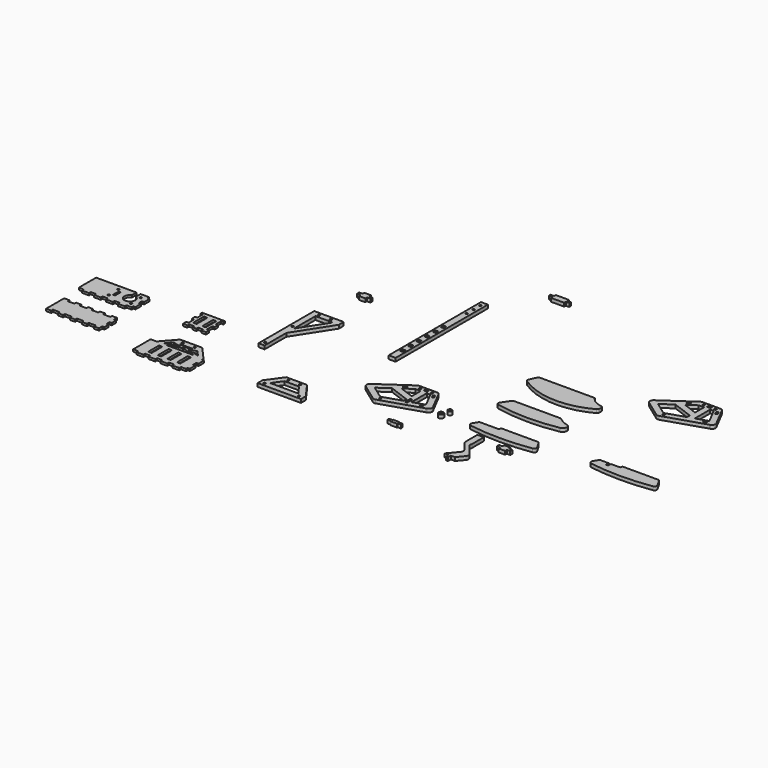
from build123d import *

# Parameters (mm, degrees)
F0_R          = 1.5
F0_W          = 3
F0_H          = 10.16
F0_W_2        = 10
F0_H_2        = 3.175
F0_W_3        = 3.175
F0_H_3        = 10
F1_DEPTH      = 3.175
F0_W_4        = 7.6
F0_H_4        = 3.1587607045
F0_H_5        = 7.5
F0_W_5        = 3.3135961294
F0_H_6        = 3
F0_W_6        = 5
F0_H_7        = 20
F0_W_7        = 6
F0_H_8        = 6
F0_W_8        = 5.2217655991
F0_W_9        = 9.1232
F2_DEPTH      = 5.08
F0_R_2        = 2.25
F0_W_10       = 5.08
F0_R_3        = 3
F0_R_4        = 3.75
F0_W_11       = 4
F0_H_9        = 5.08
F0_H_10       = 4
F0_H_11       = 5
F3_F1_R       = 5
F3_F2_R       = 5
F3_2_F1_R     = 5
F3_2_F2_R     = 5
F3_2_F3_R     = 5
F3_2_F4_R     = 5
F3_2_F5_R     = 5
F3_3_T1_DEPTH = 5.08
F3_3_T3_DEPTH = 25.1446212918
F3_3_T5_DEPTH = 19.9530496215
F3_3_T7_DEPTH = 19.9530496215
F3_4_F1_R     = 5
F3_4_F2_R     = 5
F3_4_F3_R     = 5
F3_4_F4_R     = 5
F3_4_F5_R     = 5
F4_R          = 3.5
F4_2_R        = 3.5
F4_3_R        = 3.5
F4_4_R        = 3.5
F5_R          = 1
F5_2_R        = 1
F5_3_R        = 1
F5_4_R        = 1


# Not quite as in the source:
# - a fillet or chamfer that OpenCascade refuses, or shapes differently, is made with other operations: its cross-section is extruded or revolved along the edge and cut away or added
# - a feature names something its author has since deleted; it is built from what else it names


with BuildPart() as f1:
    # F0 (on Top) → F1 (new body)
    with BuildSketch(Plane.XY):
        with BuildLine():
            Line((-51.3072787945, 47.2636158494), (-51.3072787945, 50.2636158494))
            Line((-51.3072787945, 50.2636158494), (-63.8072787945, 50.2636158494))
            Line((-63.8072787945, 50.2636158494), (-63.8072787945, 41.6798143365))
            ThreePointArc((-63.8072787945, 41.6798143365), (-60.1740292138, 38.7357518044), (-58.8072787945, 34.2636158494))
            ThreePointArc((-58.8072787945, 34.2636158494), (-71.2794147495, 27.6303662687), (-69.8072787945, 41.6798143365))
            Line((-69.8072787945, 41.6798143365), (-69.8072787945, 50.2636158494))
            Line((-69.8072787945, 50.2636158494), (-129.3072787945, 50.2636158494))
            Line((-129.3072787945, 50.2636158494), (-129.3072787945, 18.2636158494))
            Line((-129.3072787945, 18.2636158494), (-121.7072787945, 18.2636158494))
            Line((-121.7072787945, 18.2636158494), (-111.7072787945, 18.2636158494))
            Line((-111.7072787945, 18.2636158494), (-104.1072787945, 18.2636158494))
            Line((-104.1072787945, 18.2636158494), (-94.1072787945, 18.2636158494))
            Line((-94.1072787945, 18.2636158494), (-86.5072787945, 18.2636158494))
            Line((-86.5072787945, 18.2636158494), (-76.5072787945, 18.2636158494))
            Line((-76.5072787945, 18.2636158494), (-68.9072787945, 18.2636158494))
            Line((-68.9072787945, 18.2636158494), (-58.9072787945, 18.2636158494))
            Line((-58.9072787945, 18.2636158494), (-51.3072787945, 18.2636158494))
            Line((-51.3072787945, 18.2636158494), (-51.3072787945, 21.2636158494))
            Line((-51.3072787945, 21.2636158494), (-51.3072787945, 31.2636158494))
            Line((-51.3072787945, 31.2636158494), (-51.3072787945, 37.2636158494))
            Line((-51.3072787945, 37.2636158494), (-51.3072787945, 47.2636158494))
        make_face()
        with Locations((-90.9072787945, 25.3636158494)):
            Circle(F0_R, mode=Mode.SUBTRACT)
        with Locations((-85.9142787945, 34.2636158494)):
            Rectangle(F0_W, F0_H, mode=Mode.SUBTRACT)
        with Locations((-57.8072787945, 25.3636158494)):
            Circle(F0_R, mode=Mode.SUBTRACT)
        with Locations((-90.9072787945, 43.2636158494)):
            Circle(F0_R, mode=Mode.SUBTRACT)
        with Locations((-57.8072787945, 43.2636158494)):
            Circle(F0_R, mode=Mode.SUBTRACT)
        with Locations((-116.7072787945, 16.6761158494)):
            Rectangle(F0_W_2, F0_H_2)
        with Locations((-99.1072787945, 16.6761158494)):
            Rectangle(F0_W_2, F0_H_2)
        with Locations((-81.5072787945, 16.6761158494)):
            Rectangle(F0_W_2, F0_H_2)
        with Locations((-63.9072787945, 16.6761158494)):
            Rectangle(F0_W_2, F0_H_2)
        with Locations((-49.7197787945, 42.2636158494)):
            Rectangle(F0_W_3, F0_H_3)
        with Locations((-49.7197787945, 26.2636158494)):
            Rectangle(F0_W_3, F0_H_3)
    extrude(amount=F1_DEPTH)


with BuildPart() as f1b:
    # F0 (on Top) → F1, piece 2 (new body)
    with BuildSketch(Plane.XY):
        Polygon((-47.835776329, -19.1142502546), (-47.835776329, -16.1142502546), (-55.435776329, -16.1142502546), (-65.435776329, -16.1142502546), (-73.035776329, -16.1142502546), (-83.035776329, -16.1142502546), (-90.635776329, -16.1142502546), (-100.635776329, -16.1142502546), (-108.235776329, -16.1142502546), (-118.235776329, -16.1142502546), (-125.835776329, -16.1142502546), (-125.835776329, -43.1142502546), (-118.235776329, -43.1142502546), (-108.235776329, -43.1142502546), (-100.635776329, -43.1142502546), (-90.635776329, -43.1142502546), (-83.035776329, -43.1142502546), (-73.035776329, -43.1142502546), (-65.435776329, -43.1142502546), (-55.435776329, -43.1142502546), (-47.835776329, -43.1142502546), (-47.835776329, -40.1142502546), (-47.835776329, -32.6142502546), (-47.835776329, -26.6142502546), align=None)
        with Locations((-122.035776329, -14.5267502546)):
            Rectangle(F0_W_4, F0_H_2)
        with Locations((-86.835776329, -14.5348699024)):
            Rectangle(F0_W_4, F0_H_4)
        with Locations((-69.235776329, -14.5267502546)):
            Rectangle(F0_W_4, F0_H_2)
        with Locations((-51.635776329, -14.5267502546)):
            Rectangle(F0_W_4, F0_H_2)
        with Locations((-46.248276329, -22.8642502546)):
            Rectangle(F0_W_3, F0_H_5)
        with Locations((-46.248276329, -36.3642502546)):
            Rectangle(F0_W_3, F0_H_5)
        with Locations((-51.635776329, -44.7017502546)):
            Rectangle(F0_W_4, F0_H_2)
        with Locations((-69.235776329, -44.7017502546)):
            Rectangle(F0_W_4, F0_H_2)
        with Locations((-86.835776329, -44.6936306069)):
            Rectangle(F0_W_4, F0_H_4)
        with Locations((-104.435776329, -44.6936306069)):
            Rectangle(F0_W_4, F0_H_4)
        with Locations((-122.035776329, -44.7017502546)):
            Rectangle(F0_W_4, F0_H_2)
        with Locations((-104.435776329, -14.5348699024)):
            Rectangle(F0_W_4, F0_H_4)
    extrude(amount=F1_DEPTH)


with BuildPart() as f1c:
    # F0 (on Top) → F1, piece 3 (new body)
    with BuildSketch(Plane.XY):
        Polygon((26.9839958698, 26.1793102056), (23.9839958698, 26.1793102056), (20.6703997403, 26.1793102056), (20.6703997403, 23.0043102056), (26.9839958698, 23.0043102056), align=None)
        with Locations((52.6407939345, 27.6793102056)):
            Rectangle(F0_W_5, F0_H_6)
        Polygon((50.9839958698, 55.1793102056), (50.9839958698, 58.1793102056), (23.9839958698, 58.1793102056), (23.9839958698, 55.1793102056), (23.9839958698, 45.1793102056), (23.9839958698, 39.1793102056), (23.9839958698, 29.1793102056), (23.9839958698, 26.1793102056), (26.9839958698, 26.1793102056), (34.4839958698, 26.1793102056), (40.4839958698, 26.1793102056), (47.9839958698, 26.1793102056), (50.9839958698, 26.1793102056), (50.9839958698, 29.1793102056), (50.9839958698, 39.1793102056), (50.9839958698, 45.1793102056), align=None)
        with Locations((30.7339958698, 42.1793102056)):
            Rectangle(F0_W_6, F0_H_7, mode=Mode.SUBTRACT)
        with Locations((44.2339958698, 42.1793102056)):
            Rectangle(F0_W_6, F0_H_7, mode=Mode.SUBTRACT)
        with Locations((22.327197805, 27.6793102056)):
            Rectangle(F0_W_5, F0_H_6)
        with Locations((37.4839958698, 24.5918102056)):
            Rectangle(F0_W_7, F0_H_2)
        Polygon((54.2975919992, 26.1793102056), (50.9839958698, 26.1793102056), (47.9839958698, 26.1793102056), (47.9839958698, 23.0043102056), (54.2975919992, 23.0043102056), align=None)
        with Locations((22.327197805, 42.1793102056)):
            Rectangle(F0_W_5, F0_H_8)
        with Locations((22.327197805, 56.6793102056)):
            Rectangle(F0_W_5, F0_H_6)
        with Locations((52.6407939345, 42.1793102056)):
            Rectangle(F0_W_5, F0_H_8)
        with Locations((52.6407939345, 56.6793102056)):
            Rectangle(F0_W_5, F0_H_6)
    extrude(amount=F1_DEPTH)

    # F5
    f5_edges = [f1c.edges().sort_by_distance(p)[0] for p in [
        (28.233996, 52.17931, 1.5875),
        (41.733996, 52.17931, 1.5875),
        (46.733996, 52.17931, 1.5875),
        (33.233996, 52.17931, 1.5875),
        (46.733996, 32.17931, 1.5875),
        (41.733996, 32.17931, 1.5875),
        (28.233996, 32.17931, 1.5875),
        (33.233996, 32.17931, 1.5875),
    ]]
    fillet(f5_edges, radius=F5_R)


with BuildPart() as f1d:
    # F0 (on Top) → F1, piece 4 (new body)
    with BuildSketch(Plane.XY):
        with Locations((95.2578997403, -38.6101686818)):
            Rectangle(F0_W_3, F0_H_3)
        with Locations((45.8703997403, -64.1979307818)):
            Rectangle(F0_W_2, F0_H_2)
        Polygon((93.6703997403, -33.6101686818), (93.6703997403, -30.6104307818), (85.7050818996, -30.6104307818), (80.0203537034, -30.6104307818), (75.3059169408, -30.6104307818), (42.7528825399, -30.6104307818), (38.0384457773, -30.6104307818), (32.3537175811, -30.6104307818), (24.3883997403, -30.6104307818), (15.6703997403, -30.6104307818), (15.6703997403, -62.6104307818), (23.2703997403, -62.6104307818), (33.2703997403, -62.6104307818), (40.8703997403, -62.6104307818), (50.8703997403, -62.6104307818), (58.4703997403, -62.6104307818), (68.4703997403, -62.6104307818), (76.0703997403, -62.6104307818), (86.0703997403, -62.6104307818), (93.6703997403, -62.6104307818), (93.6703997403, -59.6101686818), (93.6703997403, -49.6101686818), (93.6703997403, -43.6101686818), align=None)
        Polygon((80.3059169408, -36.6104307818), (85.5276825399, -36.6104307818), (85.5276825399, -56.6104307818), (80.3059169408, -56.6104307818), (75.3059169408, -56.6104307818), (66.1827169408, -56.6104307818), (61.1827169408, -56.6104307818), (52.0595169408, -56.6104307818), (47.0595169408, -56.6104307818), (37.9363169408, -56.6104307818), (32.9363169408, -56.6104307818), (23.8131169408, -56.6104307818), (23.8131169408, -36.6104307818), (32.9363169408, -36.6104307818), (37.9363169408, -36.6104307818), (47.0595169408, -36.6104307818), (52.0595169408, -36.6104307818), (61.1827169408, -36.6104307818), (66.1827169408, -36.6104307818), (75.3059169408, -36.6104307818), align=None, mode=Mode.SUBTRACT)
        Polygon((75.3059169408, -18.8604307818), (75.3059169408, -9.8604307818), (42.7528825399, -9.8604307818), (42.7528825399, -18.8604307818), (48.4376107361, -18.8604307818), (69.6211887446, -18.8604307818), align=None)
        with Locations((50.2793997403, -14.3604307818)):
            Circle(F0_R, mode=Mode.SUBTRACT)
        with BuildLine():
            ThreePointArc((66.2793997403, -14.3604307818), (67.7793997403, -12.8604307818), (69.2793997403, -14.3604307818))
            ThreePointArc((69.2793997403, -14.3604307818), (67.7793997403, -15.8604307818), (66.2793997403, -14.3604307818))
        make_face(mode=Mode.SUBTRACT)
        with Locations((81.0703997403, -64.1979307818)):
            Rectangle(F0_W_2, F0_H_2)
        Polygon((42.7528825399, -18.8604307818), (42.7528825399, -9.8604307818), (24.3883997403, -30.6104307818), (32.3537175811, -30.6104307818), (34.1697211379, -28.5585312421), (41.644824161, -20.1124241874), align=None)
        Polygon((85.7050818996, -30.6104307818), (93.6703997403, -30.6104307818), (75.3059169408, -9.8604307818), (75.3059169408, -18.8604307818), (76.4139753197, -20.1124241874), (83.8890783427, -28.5585312421), align=None)
        with Locations((95.2578997403, -54.6101686818)):
            Rectangle(F0_W_3, F0_H_3)
        with Locations((63.4703997403, -64.1979307818)):
            Rectangle(F0_W_2, F0_H_2)
        with Locations((28.2703997403, -64.1979307818)):
            Rectangle(F0_W_2, F0_H_2)
        Polygon((75.3059169408, -20.4155445432), (75.3059169408, -18.8604307818), (69.6211887446, -18.8604307818), (59.0293997403, -21.7579196801), (64.7141279365, -23.3130334415), align=None)
        Polygon((59.0293997403, -24.8681472028), (75.3059169408, -29.3207498624), (75.3059169408, -26.2105223397), (64.7141279365, -23.3130334415), align=None)
        Polygon((42.7528825399, -29.3207498624), (59.0293997403, -24.8681472028), (53.3446715441, -23.3130334415), (42.7528825399, -26.2105223397), align=None)
        Polygon((53.3446715441, -23.3130334415), (59.0293997403, -24.8681472028), (64.7141279365, -23.3130334415), (59.0293997403, -21.7579196801), align=None)
        Polygon((48.4376107361, -18.8604307818), (42.7528825399, -18.8604307818), (42.7528825399, -20.4155445432), (53.3446715441, -23.3130334415), (59.0293997403, -21.7579196801), align=None)
        Polygon((34.1697211379, -28.5585312421), (32.3537175811, -30.6104307818), (38.0384457773, -30.6104307818), (42.7528825399, -29.3207498624), (42.7528825399, -26.2105223397), align=None)
        Polygon((80.0203537034, -30.6104307818), (85.7050818996, -30.6104307818), (83.8890783427, -28.5585312421), (75.3059169408, -26.2105223397), (75.3059169408, -29.3207498624), align=None)
        Polygon((42.7528825399, -20.4155445432), (42.7528825399, -18.8604307818), (41.644824161, -20.1124241874), align=None)
        Polygon((76.4139753197, -20.1124241874), (75.3059169408, -18.8604307818), (75.3059169408, -20.4155445432), align=None)
        with Locations((82.9167997403, -46.6104307818)):
            Rectangle(F0_W_8, F0_H_7)
        with Locations((70.7443169408, -46.6104307818)):
            Rectangle(F0_W_9, F0_H_7)
        with Locations((56.6211169408, -46.6104307818)):
            Rectangle(F0_W_9, F0_H_7)
        with Locations((42.4979169408, -46.6104307818)):
            Rectangle(F0_W_9, F0_H_7)
        with Locations((28.3747169408, -46.6104307818)):
            Rectangle(F0_W_9, F0_H_7)
    extrude(amount=F1_DEPTH)

    # F3: fillet of radius 5 on 2 edges, made by hand

    # F3_f1
    f3_f1_edges = [f1d.edges().sort_by_distance(p)[0] for p in [
        (75.3059169408, -9.8604307818, 1.5875),
    ]]
    fillet(f3_f1_edges, radius=F3_F1_R)

    # F3_f2
    f3_f2_edges = [f1d.edges().sort_by_distance(p)[0] for p in [
        (42.7528825399, -9.8604307818, 1.5875),
    ]]
    fillet(f3_f2_edges, radius=F3_F2_R)

    # F5#2
    f5_2_edges = [f1d.edges().sort_by_distance(p)[0] for p in [
        (37.936317, -36.610431, 1.5875),
        (32.936317, -36.610431, 1.5875),
        (32.936317, -56.610431, 1.5875),
        (37.936317, -56.610431, 1.5875),
        (52.059517, -56.610431, 1.5875),
        (66.182717, -56.610431, 1.5875),
        (80.305917, -56.610431, 1.5875),
        (47.059517, -56.610431, 1.5875),
        (61.182717, -56.610431, 1.5875),
        (75.305917, -56.610431, 1.5875),
        (47.059517, -36.610431, 1.5875),
        (61.182717, -36.610431, 1.5875),
        (75.305917, -36.610431, 1.5875),
        (80.305917, -36.610431, 1.5875),
        (52.059517, -36.610431, 1.5875),
        (66.182717, -36.610431, 1.5875),
    ]]
    fillet(f5_2_edges, radius=F5_2_R)


with BuildPart() as f2:
    # F0 (on Top) → F2 (new body)
    with BuildSketch(Plane.XY):
        Polygon((130.1562423062, 130.1302528989), (121.1562423062, 130.1302528989), (121.1562423062, 36.4272528989), (130.1562423062, 36.4272528989), (130.1562423062, 76.5205994248), (130.1562423062, 90.5057264181), align=None)
        with BuildLine():
            ThreePointArc((127.1562423062, 42.9272528989), (124.5955821344, 41.8665927272), (125.6562423062, 44.4272528989))
            ThreePointArc((125.6562423062, 44.4272528989), (126.716902478, 43.9879130707), (127.1562423062, 42.9272528989))
        make_face(mode=Mode.SUBTRACT)
        with BuildLine():
            ThreePointArc((125.6562423062, 92.1302528989), (124.5955821344, 94.6909130707), (127.1562423062, 93.6302528989))
            ThreePointArc((127.1562423062, 93.6302528989), (126.716902478, 92.5695927272), (125.6562423062, 92.1302528989))
        make_face(mode=Mode.SUBTRACT)
        Polygon((155.6562423062, 139.1302528989), (121.1562423062, 139.1302528989), (121.1562423062, 130.1302528989), (130.1562423062, 130.1302528989), (155.6562423062, 130.1302528989), align=None)
        with Locations((131.6562423062, 134.6302528989)):
            Circle(F0_R, mode=Mode.SUBTRACT)
        with BuildLine():
            ThreePointArc((150.6562423062, 134.6302528989), (149.1562423062, 133.1302528989), (147.6562423062, 134.6302528989))
            ThreePointArc((147.6562423062, 134.6302528989), (149.1562423062, 136.1302528989), (150.6562423062, 134.6302528989))
        make_face(mode=Mode.SUBTRACT)
        Polygon((164.6562423062, 139.1302528989), (155.6562423062, 139.1302528989), (155.6562423062, 130.1302528989), (130.1562423062, 90.5057264181), (130.1562423062, 76.5205994248), (164.6562423062, 130.1302528989), align=None)
    extrude(amount=F2_DEPTH)


with BuildPart() as f2b:
    # F0 (on Top) → F2, piece 2 (new body)
    with BuildSketch(Plane.XY):
        Polygon((193.5958625751, -32.7302958667), (182.4840346336, -32.7302958667), (182.4840346336, -41.7302958667), (246.2840346336, -41.7302958667), (246.2840346336, -32.7302958667), (235.1722066922, -32.7302958667), align=None)
        with Locations((188.9840346336, -37.2302958667)):
            Circle(F0_R, mode=Mode.SUBTRACT)
        with Locations((239.7840346336, -37.2302958667)):
            Circle(F0_R, mode=Mode.SUBTRACT)
        Polygon((199.1340346336, -9.738662824), (182.4840346336, -32.7302958667), (193.5958625751, -32.7302958667), (203.7282742106, -18.738662824), (199.1340346336, -18.738662824), align=None)
        Polygon((229.6340346336, -9.738662824), (199.1340346336, -9.738662824), (199.1340346336, -18.738662824), (203.7282742106, -18.738662824), (225.0397950567, -18.738662824), (229.6340346336, -18.738662824), align=None)
        with Locations((205.6340346336, -14.238662824)):
            Circle(F0_R, mode=Mode.SUBTRACT)
        with Locations((223.1340346336, -14.238662824)):
            Circle(F0_R, mode=Mode.SUBTRACT)
        Polygon((225.0397950567, -18.738662824), (235.1722066922, -32.7302958667), (246.2840346336, -32.7302958667), (229.6340346336, -9.738662824), (229.6340346336, -18.738662824), align=None)
    extrude(amount=F2_DEPTH)


with BuildPart() as f2c:
    # F0 (on Top) → F2, piece 3 (new body)
    with BuildSketch(Plane.XY):
        Polygon((311.7205799246, 10.2002237106), (373.359547486, 30.0294994907), (370.7162696972, 38.246083681), (367.4975760143, 37.2106288832), (350.3798130633, 31.7038390111), (347.3798130633, 30.7387380418), (347.3798130633, 27.302460951), (344.3798130633, 27.302460951), (344.3798130633, 29.7736370725), (341.3798130633, 28.8085361032), (313.6688821989, 19.8939206907), (309.0773021358, 18.4168079009), align=None)
        with Locations((316.4372015477, 16.7636158494)):
            Circle(F0_R, mode=Mode.SUBTRACT)
        with Locations((364.9868130633, 32.3820415603)):
            Circle(F0_R_2, mode=Mode.SUBTRACT)
        Polygon((361.1118909802, 69.132310951), (330.6118909802, 69.132310951), (330.6118909802, 60.132310951), (333.4160261488, 60.132310951), (341.3798130633, 60.132310951), (345.8798130633, 60.132310951), (350.3798130633, 60.132310951), (355.6356585, 60.132310951), (359.3244464957, 60.132310951), (361.1118909802, 61.0573093422), align=None)
        with Locations((337.1118909802, 64.632310951)):
            Circle(F0_R, mode=Mode.SUBTRACT)
        with Locations((345.8618909802, 64.632310951)):
            Rectangle(F0_W_10, F0_H_6, mode=Mode.SUBTRACT)
        with Locations((354.6118909802, 64.632310951)):
            Circle(F0_R, mode=Mode.SUBTRACT)
        Polygon((330.6118909802, 60.132310951), (330.6118909802, 69.132310951), (279.2187522998, 33.6640020269), (307.0271372417, 13.5885223602), (309.0773021358, 18.4168079009), (313.6688821989, 19.8939206907), (294.8239491459, 33.4984889213), (311.3826811314, 44.9262833027), (320.4336815503, 51.172713997), (333.4160261488, 60.132310951), align=None)
        Polygon((319.7851517254, 54.3702187267), (318.0811466555, 56.8393008885), (322.2621257827, 59.7247494736), (323.9661308527, 57.2556673119), align=None, mode=Mode.SUBTRACT)
        Polygon((309.0773021358, 18.4168079009), (307.0271372417, 13.5885223602), (311.7205799246, 10.2002237106), align=None)
        Polygon((350.3798130633, 60.132310951), (345.8798130633, 60.132310951), (345.8798130633, 37.462460951), (347.3798130633, 37.462460951), (347.3798130633, 30.7387380418), (350.3798130633, 31.7038390111), align=None)
        Polygon((345.8798130633, 60.132310951), (341.3798130633, 60.132310951), (341.3798130633, 43.4191280649), (341.3798130633, 33.8223073724), (341.3798130633, 28.8085361032), (344.3798130633, 29.7736370725), (344.3798130633, 37.462460951), (345.8798130633, 37.462460951), align=None)
        Polygon((380.2074692185, 32.2324781246), (361.1118909802, 69.132310951), (361.1118909802, 61.0573093422), (361.7436060326, 61.3842204224), (364.0783867233, 56.8725467721), (361.4140125204, 55.4937392776), (359.0792318297, 60.0054129279), (359.3244464957, 60.132310951), (355.6356585, 60.132310951), (367.4975760143, 37.2106288832), (370.7162696972, 38.246083681), (373.359547486, 30.0294994907), align=None)
        Polygon((341.3798130633, 43.4191280649), (320.4336815503, 51.172713997), (311.3826811314, 44.9262833027), (341.3798130633, 33.8223073724), align=None)
    extrude(amount=F2_DEPTH)

    # F3#2: fillet of radius 5 on 5 edges, made by hand

    # F3_2_f1
    f3_2_f1_edges = [f2c.edges().sort_by_distance(p)[0] for p in [
        (279.2187522998, 33.6640020269, 2.54),
    ]]
    fillet(f3_2_f1_edges, radius=F3_2_F1_R)

    # F3_2_f2
    f3_2_f2_edges = [f2c.edges().sort_by_distance(p)[0] for p in [
        (311.7205799246, 10.2002237106, 2.54),
    ]]
    fillet(f3_2_f2_edges, radius=F3_2_F2_R)

    # F3_2_f3
    f3_2_f3_edges = [f2c.edges().sort_by_distance(p)[0] for p in [
        (380.2074692185, 32.2324781246, 2.54),
    ]]
    fillet(f3_2_f3_edges, radius=F3_2_F3_R)

    # F3_2_f4
    f3_2_f4_edges = [f2c.edges().sort_by_distance(p)[0] for p in [
        (361.1118909802, 69.132310951, 2.54),
    ]]
    fillet(f3_2_f4_edges, radius=F3_2_F4_R)

    # F3_2_f5
    f3_2_f5_edges = [f2c.edges().sort_by_distance(p)[0] for p in [
        (330.6118909802, 69.132310951, 2.54),
    ]]
    fillet(f3_2_f5_edges, radius=F3_2_F5_R)


with BuildPart() as f2d:
    # F0 (on Top) → F2, piece 4 (new body)
    with BuildSketch(Plane.XY):
        with Locations((397.8557288647, 43.4133335948)):
            Circle(F0_R_3)
        with Locations((397.8557288647, 43.4133335948)):
            Circle(F0_R, mode=Mode.SUBTRACT)
    extrude(amount=F2_DEPTH)


with BuildPart() as f2e:
    # F0 (on Top) → F2, piece 5 (new body)
    with BuildSketch(Plane.XY):
        with Locations((394.295334816, 31.5429195762)):
            Circle(F0_R_4)
        with Locations((394.295334816, 31.5429195762)):
            Circle(F0_R_2, mode=Mode.SUBTRACT)
    extrude(amount=F2_DEPTH)


with BuildPart() as f2f:
    # F0 (on Top) → F2, piece 6 (new body)
    with BuildSketch(Plane.XY):
        with BuildLine():
            Line((267.2225075531, 256.5408171606), (263.6425075531, 256.5408171606))
            ThreePointArc((263.6425075531, 256.5408171606), (262.1425075531, 255.0408171606), (260.6425075531, 256.5408171606))
            Line((260.6425075531, 256.5408171606), (257.0625075531, 256.5408171606))
            Line((257.0625075531, 256.5408171606), (257.0625075531, 106.5408171606))
            Line((257.0625075531, 106.5408171606), (267.2225075531, 106.5408171606))
            Line((267.2225075531, 106.5408171606), (267.2225075531, 256.5408171606))
        make_face()
        with Locations((262.1425075531, 125.9008171606)):
            Rectangle(F0_W_11, F0_H_9, mode=Mode.SUBTRACT)
        with Locations((262.1425075531, 140.9808171606)):
            Rectangle(F0_W_11, F0_H_9, mode=Mode.SUBTRACT)
        with Locations((262.1425075531, 156.0608171606)):
            Rectangle(F0_W_11, F0_H_9, mode=Mode.SUBTRACT)
        with Locations((262.1425075531, 171.1408171606)):
            Rectangle(F0_W_11, F0_H_9, mode=Mode.SUBTRACT)
        with Locations((262.1425075531, 186.2208171606)):
            Rectangle(F0_W_11, F0_H_9, mode=Mode.SUBTRACT)
        with Locations((262.1425075531, 201.3008171606)):
            Rectangle(F0_W_11, F0_H_9, mode=Mode.SUBTRACT)
        with Locations((262.1425075531, 243.8408171606)):
            Circle(F0_R, mode=Mode.SUBTRACT)
        with BuildLine():
            ThreePointArc((260.6425075531, 256.5408171606), (262.1425075531, 258.0408171606), (263.6425075531, 256.5408171606))
            Line((263.6425075531, 256.5408171606), (267.2225075531, 256.5408171606))
            Line((267.2225075531, 256.5408171606), (267.2225075531, 276.5408171606))
            Line((267.2225075531, 276.5408171606), (257.0625075531, 276.5408171606))
            Line((257.0625075531, 276.5408171606), (257.0625075531, 256.5408171606))
            Line((257.0625075531, 256.5408171606), (260.6425075531, 256.5408171606))
        make_face()
        with Locations((262.1425075531, 269.2408171606)):
            Circle(F0_R, mode=Mode.SUBTRACT)
    extrude(amount=F2_DEPTH)


with BuildPart() as f2g:
    # F0 (on Top) → F2, piece 7 (new body)
    with BuildSketch(Plane.XY):
        with Locations((135.1781559801, 205.6855414677)):
            Rectangle(F0_W_10, F0_H_10)
        Polygon((147.2431559801, 210.7655414677), (137.7181559801, 210.7655414677), (137.7181559801, 207.6855414677), (137.7181559801, 203.6855414677), (137.7181559801, 200.6055414677), (147.2431559801, 200.6055414677), (147.2431559801, 203.6855414677), (147.2431559801, 207.6855414677), align=None)
        with Locations((149.7831559801, 205.6855414677)):
            Rectangle(F0_W_10, F0_H_10)
    extrude(amount=F2_DEPTH)


with BuildPart() as f2h:
    # F0 (on Top) → F2, piece 8 (new body)
    with BuildSketch(Plane.XY):
        with BuildLine():
            Line((508.8113546371, 171.6910898685), (426.0138634193, 171.6910898685))
            Line((426.0138634193, 171.6910898685), (419.2865788937, 157.2643816471))
            ThreePointArc((419.2865788937, 157.2643816471), (473.389794708, 138.6910267655), (529.0871487952, 151.7268320989))
            ThreePointArc((529.0871487952, 151.7268320989), (529.7864684235, 156.2130323893), (529.0944576263, 160.700365901))
            ThreePointArc((529.0944576263, 160.700365901), (517.4912728231, 163.4983205966), (508.8113546371, 171.6910898685))
        make_face()
    extrude(amount=F2_DEPTH)

    # F4
    f4_edges = [f2h.edges().sort_by_distance(p)[0] for p in [
        (419.286579, 157.264382, 2.54),
        (529.087149, 151.726832, 2.54),
        (529.094458, 160.700366, 2.54),
    ]]
    fillet(f4_edges, radius=F4_R)


with BuildPart() as f2i:
    # F0 (on Top) → F2, piece 9 (new body)
    with BuildSketch(Plane.XY):
        with BuildLine():
            Line((439.565628767, 107.5529009104), (427.5175333023, 90.3019458055))
            ThreePointArc((427.5175333023, 90.3019458055), (475.8265501408, 84.4754376444), (524.3110656738, 88.5938182473))
            ThreePointArc((524.3110656738, 88.5938182473), (528.7513573084, 92.7131814725), (528.2661914825, 98.7505614758))
            ThreePointArc((528.2661914825, 98.7505614758), (518.658357292, 101.8548541714), (510.3229284286, 107.5529009104))
            Line((510.3229284286, 107.5529009104), (439.565628767, 107.5529009104))
        make_face()
    extrude(amount=F2_DEPTH)

    # F4#2
    f4_2_edges = [f2i.edges().sort_by_distance(p)[0] for p in [
        (528.266191, 98.750561, 2.54),
        (427.517533, 90.301946, 2.54),
    ]]
    fillet(f4_2_edges, radius=F4_2_R)


with BuildPart() as f2j:
    # F0 (on Top) → F2, piece 10 (new body)
    with BuildSketch(Plane.XY):
        with BuildLine():
            Line((527.339195253, 45.3323248522), (472.048198948, 45.3323248522))
            Line((472.048198948, 45.3323248522), (471.1328413732, 41.9161638759))
            Line((471.1328413732, 41.9161638759), (442.339195253, 41.9161638759))
            Line((442.339195253, 41.9161638759), (435.1845085621, 29.5238830149))
            ThreePointArc((435.1845085621, 29.5238830149), (485.8253559827, 25.3323248522), (536.4662034032, 29.5238830149))
            Line((536.4662034032, 29.5238830149), (527.339195253, 45.3323248522))
        make_face()
    extrude(amount=F2_DEPTH)

    # F4#3
    f4_3_edges = [f2j.edges().sort_by_distance(p)[0] for p in [
        (435.184509, 29.523883, 2.54),
        (442.339195, 41.916164, 2.54),
        (527.339195, 45.332325, 2.54),
        (536.466203, 29.523883, 2.54),
    ]]
    fillet(f4_3_edges, radius=F4_3_R)

    # F5#3
    f5_3_edges = [f2j.edges().sort_by_distance(p)[0] for p in [
        (471.132841, 41.916164, 2.54),
        (472.048199, 45.332325, 2.54),
    ]]
    fillet(f5_3_edges, radius=F5_3_R)


with BuildPart() as f2k:
    # F0 (on Top) → F2, piece 11 (new body)
    with BuildSketch(Plane.XY):
        Polygon((474.8192946437, -26.5522380743), (460.1350510981, -44.0522380743), (466.1350510981, -44.0522380743), (469.1350510981, -44.0522380743), (475.1350510981, -44.0522380743), (485.9345713908, -31.1818709671), (469.1936320931, -9.3646541091), (461.630797609, -9.3646541091), align=None)
        with Locations((467.6350510981, -46.5522380743)):
            Rectangle(F0_W, F0_H_11)
        Polygon((460.6497148511, -9.3646541091), (461.630797609, -9.3646541091), (469.1936320931, -9.3646541091), (470.1747148511, -9.3646541091), (470.1747148511, 15.6353458909), (465.4122148511, 15.6353458909), (460.6497148511, 15.6353458909), align=None)
    extrude(amount=F2_DEPTH)

    # F3#3: fillet of radius 5 on 4 edges, made by hand

    # F3_3_s2 → F3_3_t1 (join)
    with BuildSketch(Plane.XY):
        with BuildLine():
            ThreePointArc((472.3763811377, -23.3685712096), (473.4084245716, -26.5214527798), (472.2398366518, -29.6263164031))
            Line((472.2398366518, -29.6263164031), (474.8192946437, -26.5522380743))
            Line((474.8192946437, -26.5522380743), (472.3763811377, -23.3685712096))
        make_face()
    extrude(amount=F3_3_T1_DEPTH)

    # F3_3_s4 → F3_3_t3 (cut)
    with BuildSketch(Plane.XY.offset(-10.0323106459)):
        with BuildLine():
            ThreePointArc((483.3551133989, -34.2559492959), (484.5237013188, -31.1510856727), (483.4916578848, -27.9982041024))
            Line((483.4916578848, -27.9982041024), (485.9345713908, -31.1818709671))
            Line((485.9345713908, -31.1818709671), (483.3551133989, -34.2559492959))
        make_face()
    extrude(amount=F3_3_T3_DEPTH, mode=Mode.SUBTRACT)

    # F3_3_s6 → F3_3_t5 (cut)
    with BuildSketch(Plane.XY.offset(-7.4365248107)):
        with BuildLine():
            ThreePointArc((470.1747148511, -6.3900441848), (469.9231138555, -7.9561562163), (469.1936320931, -9.3646541091))
            Line((469.1936320931, -9.3646541091), (470.1747148511, -9.3646541091))
            Line((470.1747148511, -9.3646541091), (470.1747148511, -6.3900441848))
        make_face()
    extrude(amount=F3_3_T5_DEPTH, mode=Mode.SUBTRACT)

    # F3_3_s8 → F3_3_t7 (cut)
    with BuildSketch(Plane.XY.offset(-7.4365248107)):
        with BuildLine():
            ThreePointArc((461.630797609, -9.3646541091), (460.9013158466, -7.9561562163), (460.6497148511, -6.3900441848))
            Line((460.6497148511, -6.3900441848), (460.6497148511, -9.3646541091))
            Line((460.6497148511, -9.3646541091), (461.630797609, -9.3646541091))
        make_face()
    extrude(amount=F3_3_T7_DEPTH, mode=Mode.SUBTRACT)


with BuildPart() as f2l:
    # F0 (on Top) → F2, piece 12 (new body)
    with BuildSketch(Plane.XY):
        with BuildLine():
            Line((694.5588042752, 58.1520918505), (640.47416185, 58.1520918505))
            Line((640.47416185, 58.1520918505), (639.5588042752, 54.7359308742))
            Line((639.5588042752, 54.7359308742), (626.0588042752, 54.7359308742))
            Line((626.0588042752, 54.7359308742), (626.0588042752, 49.7359308742))
            Line((626.0588042752, 49.7359308742), (623.0588042752, 49.7359308742))
            Line((623.0588042752, 49.7359308742), (623.0588042752, 54.7359308742))
            Line((623.0588042752, 54.7359308742), (609.5588042752, 54.7359308742))
            Line((609.5588042752, 54.7359308742), (602.4041175842, 42.3436500132))
            ThreePointArc((602.4041175842, 42.3436500132), (653.0449650048, 38.1520918505), (703.6858124254, 42.3436500132))
            Line((703.6858124254, 42.3436500132), (694.5588042752, 58.1520918505))
        make_face()
    extrude(amount=F2_DEPTH)

    # F4#4
    f4_4_edges = [f2l.edges().sort_by_distance(p)[0] for p in [
        (602.404118, 42.34365, 2.54),
        (703.685812, 42.34365, 2.54),
    ]]
    fillet(f4_4_edges, radius=F4_4_R)

    # F5#4
    f5_4_edges = [f2l.edges().sort_by_distance(p)[0] for p in [
        (639.558804, 54.735931, 2.54),
        (640.474162, 58.152092, 2.54),
    ]]
    fillet(f5_4_edges, radius=F5_4_R)


with BuildPart() as f2m:
    # F0 (on Top) → F2, piece 13 (new body)
    with BuildSketch(Plane.XY):
        with Locations((358.7300402737, -18.1356719136)):
            Rectangle(F0_W_10, F0_H_6)
        Polygon((370.7950402737, -15.6356719136), (361.2700402737, -15.6356719136), (361.2700402737, -16.6356719136), (361.2700402737, -19.6356719136), (361.2700402737, -20.6356719136), (370.7950402737, -20.6356719136), (370.7950402737, -19.6356719136), (370.7950402737, -16.6356719136), align=None)
        with Locations((373.3350402737, -18.1356719136)):
            Rectangle(F0_W_10, F0_H_6)
    extrude(amount=F2_DEPTH)


with BuildPart() as f2n:
    # F0 (on Top) → F2, piece 14 (new body)
    with BuildSketch(Plane.XY):
        Polygon((510.4926814079, 11.3272481728), (510.4926814079, 14.4072481728), (500.9676814079, 14.4072481728), (500.9676814079, 11.3272481728), (500.9676814079, 7.3272481728), (500.9676814079, 4.2472481728), (510.4926814079, 4.2472481728), (510.4926814079, 7.3272481728), align=None)
        with Locations((513.0326814079, 9.3272481728)):
            Rectangle(F0_W_10, F0_H_10)
        with Locations((498.4276814079, 9.3272481728)):
            Rectangle(F0_W_10, F0_H_10)
    extrude(amount=F2_DEPTH)


with BuildPart() as f2o:
    # F0 (on Top) → F2, piece 15 (new body)
    with BuildSketch(Plane.XY):
        Polygon((332.9450486279, 344.0582420826), (313.2600486279, 344.0582420826), (313.2600486279, 341.0582420826), (313.2600486279, 338.0582420826), (313.2600486279, 335.0582420826), (332.9450486279, 335.0582420826), (332.9450486279, 338.0582420826), (332.9450486279, 341.0582420826), align=None)
        with Locations((310.7200486279, 339.5582420826)):
            Rectangle(F0_W_10, F0_H_6)
        with Locations((335.4850486279, 339.5582420826)):
            Rectangle(F0_W_10, F0_H_6)
    extrude(amount=F2_DEPTH)


with BuildPart() as f2p:
    # F0 (on Top) → F2, piece 16 (new body)
    with BuildSketch(Plane.XY):
        Polygon((641.2618259376, 241.1788615151), (610.7618259376, 241.1788615151), (610.7618259376, 232.1788615151), (613.5659611062, 232.1788615151), (621.5297480207, 232.1788615151), (626.0297480207, 232.1788615151), (630.5297480207, 232.1788615151), (635.7855934574, 232.1788615151), (639.474381453, 232.1788615151), (641.2618259376, 233.1038599063), align=None)
        with Locations((617.2618259376, 236.6788615151)):
            Circle(F0_R, mode=Mode.SUBTRACT)
        with Locations((626.0118259376, 236.6788615151)):
            Rectangle(F0_W_10, F0_H_6, mode=Mode.SUBTRACT)
        with Locations((634.7618259376, 236.6788615151)):
            Circle(F0_R, mode=Mode.SUBTRACT)
        Polygon((610.7618259376, 232.1788615151), (610.7618259376, 241.1788615151), (559.3686872572, 205.710552591), (587.1770721991, 185.6350729243), (589.2272370932, 190.4633584649), (593.8188171563, 191.9404712548), (574.9738841033, 205.5450394854), (591.5326160887, 216.9728338667), (600.5836165077, 223.2192645611), (613.5659611062, 232.1788615151), align=None)
        Polygon((599.9350866828, 226.4167692908), (598.2310816129, 228.8858514526), (602.4120607401, 231.7713000377), (604.1160658101, 229.3022178759), align=None, mode=Mode.SUBTRACT)
        Polygon((621.5297480207, 215.4656786289), (600.5836165077, 223.2192645611), (591.5326160887, 216.9728338667), (621.5297480207, 205.8688579365), align=None)
        Polygon((630.5297480207, 232.1788615151), (626.0297480207, 232.1788615151), (626.0297480207, 202.3027381212), (630.5297480207, 203.7503895752), align=None)
        Polygon((626.0297480207, 232.1788615151), (621.5297480207, 232.1788615151), (621.5297480207, 215.4656786289), (621.5297480207, 205.8688579365), (621.5297480207, 200.8550866673), (626.0297480207, 202.3027381212), align=None)
        Polygon((660.3574041758, 204.2790286886), (641.2618259376, 241.1788615151), (641.2618259376, 233.1038599063), (641.8935409899, 233.4307709864), (644.2283216806, 228.9190973362), (641.5639474778, 227.5402898417), (639.229166787, 232.0519634919), (639.474381453, 232.1788615151), (635.7855934574, 232.1788615151), (647.6475109717, 209.2571794473), (650.8662046546, 210.292634245), (653.5094824434, 202.0760500547), align=None)
        Polygon((591.870514882, 182.2467742746), (653.5094824434, 202.0760500547), (650.8662046546, 210.292634245), (647.6475109717, 209.2571794473), (630.5297480207, 203.7503895752), (626.0297480207, 202.3027381212), (621.5297480207, 200.8550866673), (593.8188171563, 191.9404712548), (589.2272370932, 190.4633584649), align=None)
        with Locations((596.5871365051, 188.8101664134)):
            Circle(F0_R, mode=Mode.SUBTRACT)
        with Locations((645.1367480207, 204.4285921244)):
            Circle(F0_R_2, mode=Mode.SUBTRACT)
        Polygon((589.2272370932, 190.4633584649), (587.1770721991, 185.6350729243), (591.870514882, 182.2467742746), align=None)
    extrude(amount=F2_DEPTH)

    # F3#4: fillet of radius 5 on 5 edges, made by hand

    # F3_4_f1
    f3_4_f1_edges = [f2p.edges().sort_by_distance(p)[0] for p in [
        (641.2618259376, 241.1788615151, 2.54),
    ]]
    fillet(f3_4_f1_edges, radius=F3_4_F1_R)

    # F3_4_f2
    f3_4_f2_edges = [f2p.edges().sort_by_distance(p)[0] for p in [
        (610.7618259376, 241.1788615151, 2.54),
    ]]
    fillet(f3_4_f2_edges, radius=F3_4_F2_R)

    # F3_4_f3
    f3_4_f3_edges = [f2p.edges().sort_by_distance(p)[0] for p in [
        (559.3686872572, 205.710552591, 2.54),
    ]]
    fillet(f3_4_f3_edges, radius=F3_4_F3_R)

    # F3_4_f4
    f3_4_f4_edges = [f2p.edges().sort_by_distance(p)[0] for p in [
        (591.870514882, 182.2467742746, 2.54),
    ]]
    fillet(f3_4_f4_edges, radius=F3_4_F4_R)

    # F3_4_f5
    f3_4_f5_edges = [f2p.edges().sort_by_distance(p)[0] for p in [
        (660.3574041758, 204.2790286886, 2.54),
    ]]
    fillet(f3_4_f5_edges, radius=F3_4_F5_R)


solid = Compound([f1.part, f1b.part, f1c.part, f1d.part, f2.part, f2b.part, f2c.part, f2d.part, f2e.part, f2f.part, f2g.part, f2h.part, f2i.part, f2j.part, f2k.part, f2l.part, f2m.part, f2n.part, f2o.part, f2p.part])
